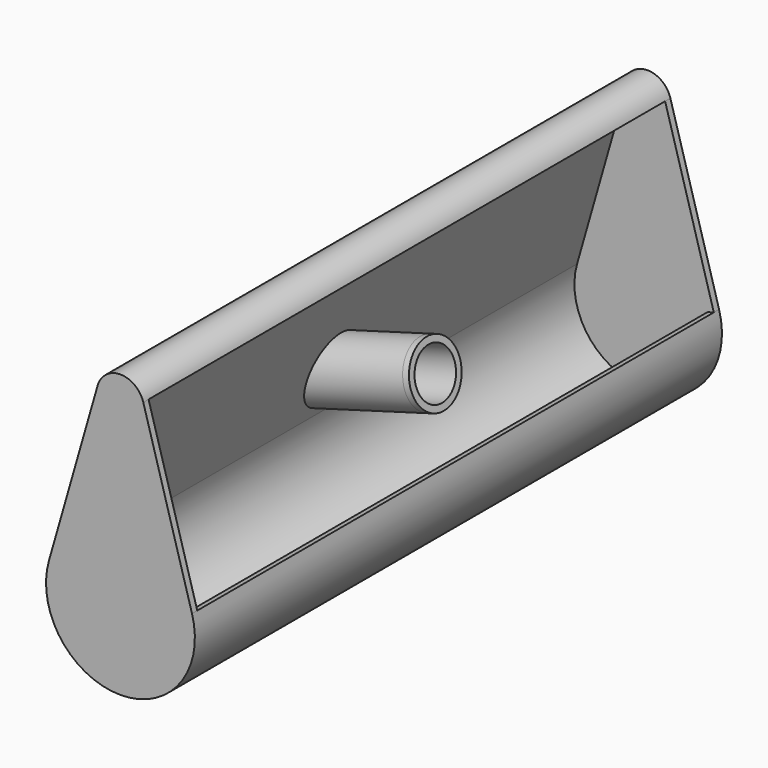
from build123d import *

# Parameters (mm, degrees)
F1_DEPTH = 254
F2_R     = 9.4654470454
F3_DEPTH = 64.1706123384
F4_T     = -2.54


# Not quite as in the source:
# - a shell that OpenCascade refuses in one call is made with other operations: the cavity is built on its own and cut out


with BuildPart() as f1:
    # F0 (on Front) → F1 (new body)
    with BuildSketch(Plane.XZ):
        with BuildLine():
            Line((-8.8068979187, 65.0390158129), (-27.5814907687, -0.52515852))
            ThreePointArc((-27.5814907687, -0.52515852), (0, -37.1132800896), (27.5814907687, -0.52515852))
            Line((27.5814907687, -0.52515852), (8.8068979187, 65.0390158129))
            ThreePointArc((8.8068979187, 65.0390158129), (0, 71.6779839596), (-8.8068979187, 65.0390158129))
        make_face()
    extrude(amount=F1_DEPTH)

    # F2 (on face) → F3 (cut, through all)
    with BuildSketch(Plane(origin=(25.3522532018, 0, 7.2597304326), x_dir=(0, 1, 0), z_dir=(0.961361214, 0, 0.2752900583))):
        with Locations((-127, 20.2662516385)):
            Circle(F2_R)
    extrude(amount=-F3_DEPTH, mode=Mode.SUBTRACT)

    # F4: a shell. OpenCascade refuses it in one call, so the cavity is built on its own and cut out:
    # the body offset inwards by the wall thickness, plus a prism from it out through each open face.
    f4_core = offset(f1.part, amount=F4_T, mode=Mode.PRIVATE)
    f4_exits = [f4_core.faces().sort_by_distance(p)[0] for p in [
        (24.429127, -127, 1.256817),
    ]]
    add(f4_core, mode=Mode.SUBTRACT)
    extrude(f4_exits, amount=-F4_T, mode=Mode.SUBTRACT)


solid = f1.part
